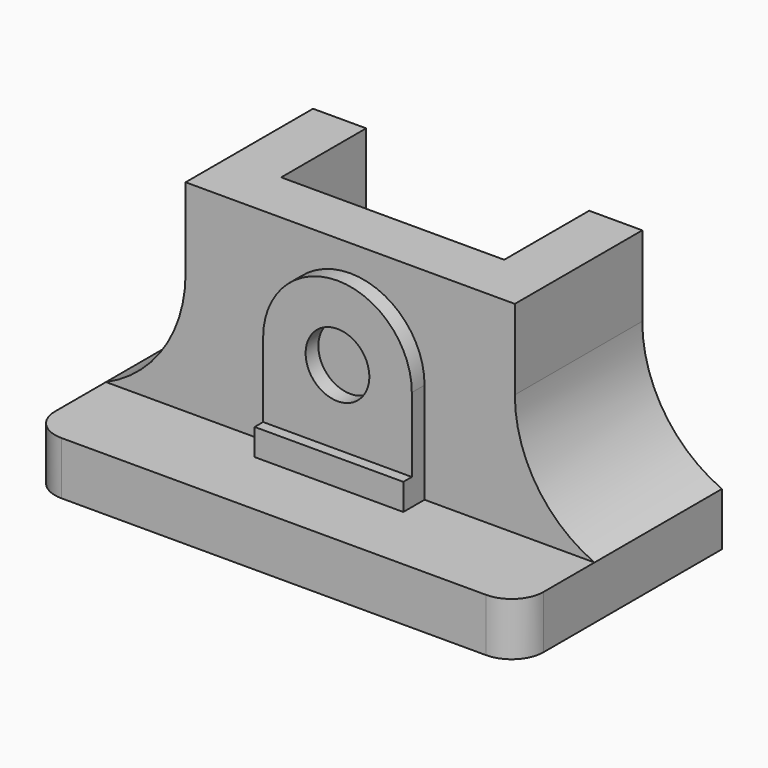
from build123d import *

# Parameters (mm, degrees)
F0_W        = 15
F0_H        = 30
F1_DEPTH    = 48
F2_DEPTH    = 10
F3_W        = 15
F3_H        = 30
F4_DEPTH    = 38
F5_T1_DEPTH = 30
F7_DEPTH    = 3
F8_W        = 28
F8_H        = 5
F9_DEPTH    = 2
F10_R       = 6


# Not quite as in the source:
# - a fillet or chamfer that OpenCascade refuses, or shapes differently, is made with other operations: its cross-section is extruded or revolved along the edge and cut away or added


with BuildPart() as f1:
    # F0 (on Top) → F1 (new body)
    with BuildSketch(Plane.XY):
        Polygon((21, 10), (0, 10), (-21, 10), (-21, 30), (-31, 30), (-31, 0), (31, 0), (31, 30), (21, 30), align=None)
        with Locations((38.5, 15)):
            Rectangle(F0_W, F0_H)
        with Locations((-38.5, 15)):
            Rectangle(F0_W, F0_H)
    extrude(amount=F1_DEPTH)

    # F0 (on Top) → F2 (join)
    with BuildSketch(Plane.XY):
        Polygon((31, 0), (-31, 0), (-46, 0), (-46, -18), (46, -18), (46, 0), align=None)
    extrude(amount=F2_DEPTH)

    # F3 (on face) → F4 (cut)
    with BuildSketch(Plane.XY.offset(48)):
        with Locations((-38.5, 15)):
            Rectangle(F3_W, F3_H)
        with Locations((38.5, 15)):
            Rectangle(F3_W, F3_H)
    extrude(amount=-F4_DEPTH, mode=Mode.SUBTRACT)

    # F5: fillet of radius 25 on 2 edges, made by hand

    # F5_s2 → F5_t1 (join)
    with BuildSketch(Plane.XZ.offset(-30)):
        with BuildLine():
            ThreePointArc((46, 10), (35.0834993366, 19.2198145372), (31, 32.9128784748))
            Line((31, 32.9128784748), (31, 10))
            Line((31, 10), (46, 10))
        make_face()
        with BuildLine():
            ThreePointArc((-46, 10), (-35.0834993366, 19.2198145372), (-31, 32.9128784748))
            Line((-31, 32.9128784748), (-31, 10))
            Line((-31, 10), (-46, 10))
        make_face()
    extrude(amount=F5_T1_DEPTH)

    # F6 (on face) → F7 (join)
    with BuildSketch(Plane.XZ):
        with BuildLine():
            Line((-14, 29), (-14, 10))
            Line((-14, 10), (14, 10))
            Line((14, 10), (14, 29))
            Line((14, 29), (6, 29))
            ThreePointArc((6, 29), (0, 23), (-6, 29))
            Line((-6, 29), (-14, 29))
        make_face()
        with BuildLine():
            ThreePointArc((14, 29), (0, 43), (-14, 29))
            Line((-14, 29), (-6, 29))
            ThreePointArc((-6, 29), (0, 35), (6, 29))
            Line((6, 29), (14, 29))
        make_face()
    extrude(amount=F7_DEPTH)

    # F8 (on face) → F9 (join)
    with BuildSketch(Plane.XZ.offset(3)):
        with Locations((0, 12.5)):
            Rectangle(F8_W, F8_H)
    extrude(amount=F9_DEPTH)

    # F10
    f10_edges = [f1.edges().sort_by_distance(p)[0] for p in [
        (46, -18, 5),
        (-46, -18, 5),
    ]]
    fillet(f10_edges, radius=F10_R)


solid = f1.part
